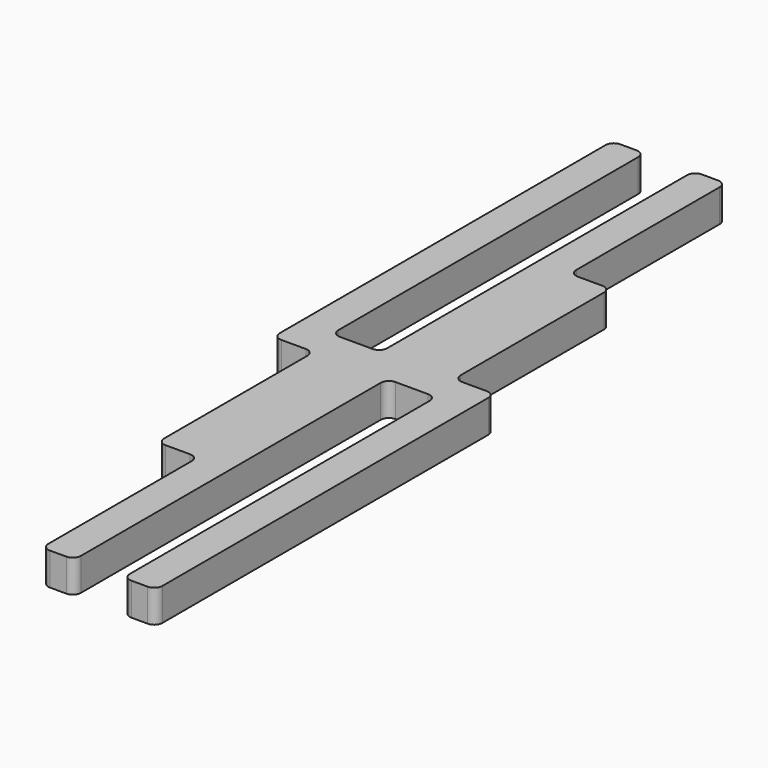
from build123d import *

# Parameters (mm, degrees)
F0_W     = 2.5
F0_H     = 12
F1_DEPTH = 2
F2_R     = 0.5


with BuildPart() as f1:
    # F0 (on Top) → F1 (new body)
    with BuildSketch(Plane.XY):
        Polygon((-1, -13), (-1, -25), (1, -25), (1, -1), (1, 1), (1, 13), (1, 25), (-1, 25), (-1, 1), (-1, -1), align=None)
        with Locations((-2.25, -7)):
            Rectangle(F0_W, F0_H)
        Polygon((1, 1), (1, -1), (4, -1), (4, -25), (6, -25), (6, 1), (3.5, 1), align=None)
        Polygon((-3.5, -1), (-1, -1), (-1, 1), (-4, 1), (-4, 25), (-6, 25), (-6, -1), align=None)
        with Locations((2.25, 7)):
            Rectangle(F0_W, F0_H)
    extrude(amount=F1_DEPTH)

    # F2
    f2_edges = [f1.edges().sort_by_distance(p)[0] for p in [
        (-1, -25, 1),
        (-1, 1, 1),
        (-6, -1, 1),
        (1, -25, 1),
        (4, -25, 1),
        (6, -25, 1),
        (1, -1, 1),
        (4, -1, 1),
        (6, 1, 1),
        (-4, 1, 1),
        (-6, 25, 1),
        (-4, 25, 1),
        (-1, 25, 1),
        (1, 25, 1),
        (3.5, 13, 1),
        (-3.5, -13, 1),
        (-3.5, -1, 1),
        (3.5, 1, 1),
        (-1, -13, 1),
        (1, 13, 1),
    ]]
    fillet(f2_edges, radius=F2_R)


solid = f1.part
